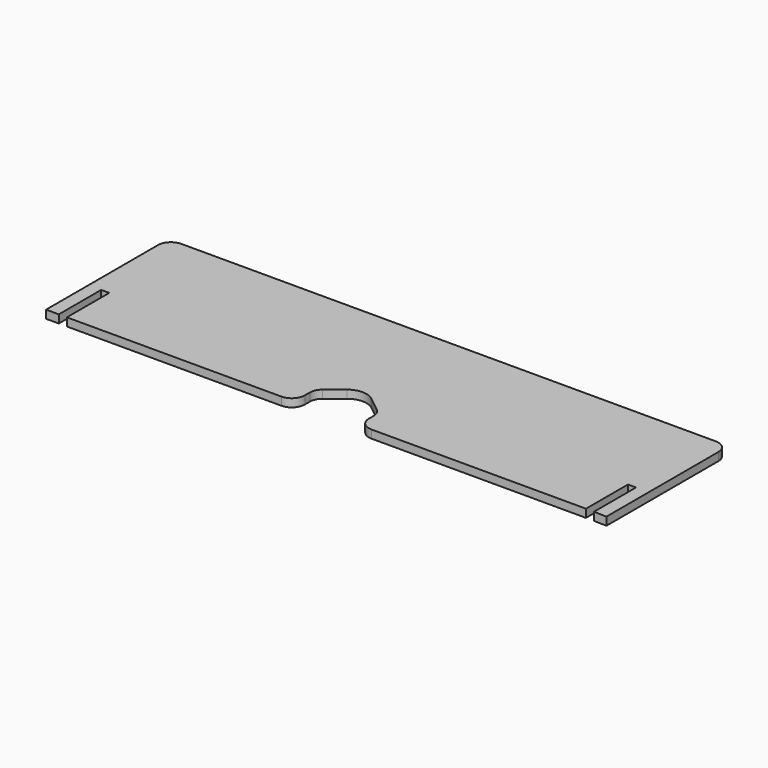
from build123d import *

# Parameters (mm, degrees)
F1_DEPTH = 3.175


# Not quite as in the source:
# - a length typed as a fraction of an inch, garbled in the dataset ("3 / 203.2 mm" for 3/8 in), is restored


with BuildPart() as f1:
    # F0 (on Top) → F1 (new body)
    with BuildSketch(Plane.XY):
        with BuildLine():
            ThreePointArc((110, 24.92), (108.5121024484, 28.5121024484), (104.92, 30))
            Line((104.92, 30), (-104.92, 30))
            ThreePointArc((-104.92, 30), (-108.5121024484, 28.5121024484), (-110, 24.92))
            Line((-110, 24.92), (-110, -30))
            Line((-110, -30), (-105, -30))
            Line((-105, -30), (-105, -9.2280227691))
            Line((-105, -9.2280227691), (-101.825, -9.2280227691))
            Line((-101.825, -9.2280227691), (-101.825, -30))
            Line((-101.825, -30), (-17.58, -30))
            ThreePointArc((-17.58, -30), (-13.9878975516, -28.5121024484), (-12.5, -24.92))
            Line((-12.5, -24.92), (-12.5, -22.4415742252))
            ThreePointArc((-12.5, -22.4415742252), (-11.9986204404, -20.2409754743), (-10.5934508416, -18.4747606733))
            Line((-10.5934508416, -18.4747606733), (-4.7601762624, -13.8081410099))
            ThreePointArc((-4.7601762624, -13.8081410099), (0, -12.1383613378), (4.7601762624, -13.8081410099))
            Line((4.7601762624, -13.8081410099), (10.5934508416, -18.4747606733))
            ThreePointArc((10.5934508416, -18.4747606733), (11.9986204404, -20.2409754743), (12.5, -22.4415742252))
            Line((12.5, -22.4415742252), (12.5, -24.7250270788))
            ThreePointArc((12.5, -24.7250270788), (13.9878975516, -28.3171295272), (17.58, -29.8050270788))
            Line((17.58, -29.8050270788), (101.825, -29.8050270788))
            Line((101.825, -29.8050270788), (101.825, -9.2280227691))
            Line((101.825, -9.2280227691), (105, -9.2280227691))
            Line((105, -9.2280227691), (105, -29.8050270788))
            Line((105, -29.8050270788), (110, -30))
            Line((110, -30), (110, 24.92))
        make_face()
    extrude(amount=F1_DEPTH)


solid = f1.part
